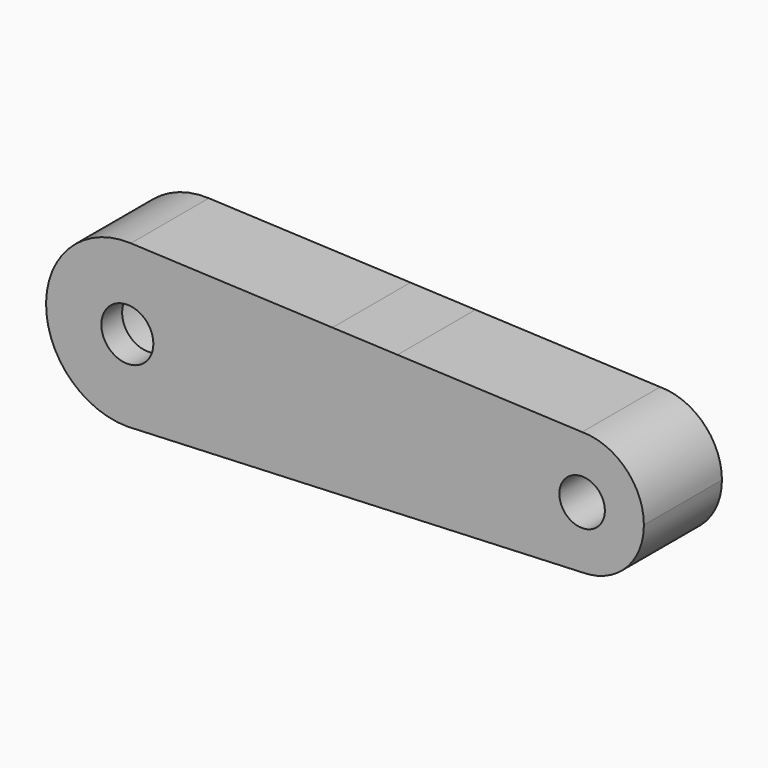
from build123d import *

# Parameters (mm, degrees)
F0_R     = 4.445
F1_DEPTH = 19.05
F3_DEPTH = 13.97
F4_R     = 5.08
F5_DEPTH = 5.08


with BuildPart() as f1:
    # F0 (on Front) → F1 (new body)
    with BuildSketch(Plane.XZ):
        with BuildLine():
            ThreePointArc((-124.9322268395, 28.7639294598), (-130.4980059639, 35.017678352), (-138.4710976488, 37.5705358593))
            ThreePointArc((-138.4710976488, 37.5705358593), (-155.0254015346, 22.0518028606), (-139.1540765762, 5.8352343242))
            Line((-139.1540765762, 5.8352343242), (-137.7946125004, 5.8935506507))
            ThreePointArc((-137.7946125004, 5.8935506507), (-130.1034423833, 8.6679321614), (-124.8131018813, 14.9019988847))
            Line((-124.8131018813, 14.9019988847), (-133.3336122029, 14.1704850261))
            ThreePointArc((-133.3336122029, 14.1704850261), (-148.6790765762, 21.7102343242), (-133.3336122029, 29.2499836224))
            Line((-133.3336122029, 29.2499836224), (-124.9322268395, 28.7639294598))
        make_face()
        with BuildLine():
            Line((-99.1008544222, 34.8894799677), (-99.1008544222, 35.8751666308))
            Line((-99.1008544222, 35.8751666308), (-138.4710976488, 37.5705358593))
            ThreePointArc((-138.4710976488, 37.5705358593), (-130.4980059639, 35.017678352), (-124.9322268395, 28.7639294598))
            Line((-124.9322268395, 28.7639294598), (-110.4319389367, 27.9250290893))
            ThreePointArc((-110.4319389367, 27.9250290893), (-105.7509869831, 33.0091720577), (-99.1008544222, 34.8894799677))
        make_face()
        with BuildLine():
            Line((-137.7946125004, 5.8935506507), (-99.0179549294, 7.5569357044))
            Line((-99.0179549294, 7.5569357044), (-99.1008544222, 9.4894799677))
            ThreePointArc((-99.1008544222, 9.4894799677), (-105.6044119808, 11.2810548255), (-110.273070294, 16.1503084588))
            Line((-110.273070294, 16.1503084588), (-124.8131018813, 14.9019988847))
            ThreePointArc((-124.8131018813, 14.9019988847), (-130.1034423833, 8.6679321614), (-137.7946125004, 5.8935506507))
        make_face()
        with BuildLine():
            ThreePointArc((-99.1008544222, 9.4894799677), (-96.8524942518, 9.6900849205), (-94.6751627721, 10.2855624017))
            ThreePointArc((-94.6751627721, 10.2855624017), (-88.6726167006, 14.9409036921), (-86.4008544222, 22.1894799677))
            Line((-86.4008544222, 22.1894799677), (-94.0208544222, 22.1894799677))
            ThreePointArc((-94.0208544222, 22.1894799677), (-95.5087519738, 18.5973775193), (-99.1008544222, 17.1094799677))
            Line((-99.1008544222, 17.1094799677), (-110.273070294, 16.1503084588))
            ThreePointArc((-110.273070294, 16.1503084588), (-105.6044119808, 11.2810548255), (-99.1008544222, 9.4894799677))
        make_face()
        with BuildLine():
            ThreePointArc((-86.4008544222, 22.1894799677), (-88.0348602906, 28.4211550137), (-92.5164093638, 33.0492720132))
            ThreePointArc((-92.5164093638, 33.0492720132), (-95.6824746143, 34.4207791419), (-99.1008544222, 34.8894799677))
            ThreePointArc((-99.1008544222, 34.8894799677), (-105.7509869831, 33.0091720577), (-110.4319389367, 27.9250290893))
            Line((-110.4319389367, 27.9250290893), (-99.1008544222, 27.2694799677))
            ThreePointArc((-99.1008544222, 27.2694799677), (-95.5087519738, 25.7815824161), (-94.0208544222, 22.1894799677))
            Line((-94.0208544222, 22.1894799677), (-86.4008544222, 22.1894799677))
        make_face()
        with BuildLine():
            Line((-99.0179549294, 7.5569357044), (-87.6442336226, 8.0448291746))
            Line((-87.6442336226, 8.0448291746), (-87.7530907655, 10.5824954495))
            Line((-87.7530907655, 10.5824954495), (-94.6751627721, 10.2855624017))
            ThreePointArc((-94.6751627721, 10.2855624017), (-96.8524942518, 9.6900849205), (-99.1008544222, 9.4894799677))
            Line((-99.1008544222, 9.4894799677), (-99.0179549294, 7.5569357044))
        make_face()
        with BuildLine():
            Line((-86.5101311345, 32.7906284679), (-86.4008544222, 35.3282767099))
            Line((-86.4008544222, 35.3282767099), (-99.1008544222, 35.8751666308))
            Line((-99.1008544222, 35.8751666308), (-99.1008544222, 34.8894799677))
            ThreePointArc((-99.1008544222, 34.8894799677), (-95.6824746143, 34.4207791419), (-92.5164093638, 33.0492720132))
            Line((-92.5164093638, 33.0492720132), (-86.5101311345, 32.7906284679))
        make_face()
        with BuildLine():
            ThreePointArc((-57.3392350777, 31.5344655517), (-54.0123637648, 33.2013955962), (-50.3357569569, 33.7752343242))
            Line((-50.3357569569, 33.7752343242), (-86.4008544222, 35.3282767099))
            Line((-86.4008544222, 35.3282767099), (-86.5101311345, 32.7906284679))
            Line((-86.5101311345, 32.7906284679), (-57.3392350777, 31.5344655517))
        make_face()
        with BuildLine():
            Line((-87.6442336226, 8.0448291746), (-50.3357569569, 9.6452343242))
            ThreePointArc((-50.3357569569, 9.6452343242), (-54.0132473827, 10.2193558039), (-57.3407458906, 11.8870802972))
            Line((-57.3407458906, 11.8870802972), (-87.7530907655, 10.5824954495))
            Line((-87.7530907655, 10.5824954495), (-87.6442336226, 8.0448291746))
        make_face()
        with BuildLine():
            ThreePointArc((-50.3357569569, 9.6452343242), (-41.8045136419, 13.1789910092), (-38.2707569569, 21.7102343242))
            ThreePointArc((-38.2707569569, 21.7102343242), (-41.8045136419, 30.2414776392), (-50.3357569569, 33.7752343242))
            ThreePointArc((-50.3357569569, 33.7752343242), (-54.0123637648, 33.2013955962), (-57.3392350777, 31.5344655517))
            ThreePointArc((-57.3392350777, 31.5344655517), (-62.4007569212, 21.7111620791), (-57.3407458906, 11.8870802972))
            ThreePointArc((-57.3407458906, 11.8870802972), (-54.0132473827, 10.2193558039), (-50.3357569569, 9.6452343242))
        make_face()
        with Locations((-50.3357569569, 21.7102343242)):
            Circle(F0_R, mode=Mode.SUBTRACT)
    extrude(amount=F1_DEPTH)

    # F2 (on face) → F3 (join)
    with BuildSketch(Plane.XZ.offset(19.05)):
        with BuildLine():
            ThreePointArc((-86.4008544222, 22.1894799677), (-88.6726167006, 14.9409036921), (-94.6751627721, 10.2855624017))
            Line((-94.6751627721, 10.2855624017), (-57.3407458906, 11.8870802972))
            ThreePointArc((-57.3407458906, 11.8870802972), (-62.4007569212, 21.7111620791), (-57.3392350777, 31.5344655517))
            Line((-57.3392350777, 31.5344655517), (-92.5164093638, 33.0492720132))
            ThreePointArc((-92.5164093638, 33.0492720132), (-88.0348602906, 28.4211550137), (-86.4008544222, 22.1894799677))
        make_face()
        with BuildLine():
            Line((-57.3407458906, 11.8870802972), (-94.6751627721, 10.2855624017))
            ThreePointArc((-94.6751627721, 10.2855624017), (-103.5704974557, 10.301995324), (-110.273070294, 16.1503084588))
            Line((-110.273070294, 16.1503084588), (-133.3336122029, 14.1704850261))
            ThreePointArc((-133.3336122029, 14.1704850261), (-148.6790765762, 21.7102343242), (-133.3336122029, 29.2499836224))
            Line((-133.3336122029, 29.2499836224), (-110.4319389367, 27.9250290893))
            ThreePointArc((-110.4319389367, 27.9250290893), (-102.5932909524, 34.3998397938), (-92.5164093638, 33.0492720132))
            Line((-92.5164093638, 33.0492720132), (-57.3392350777, 31.5344655517))
            ThreePointArc((-57.3392350777, 31.5344655517), (-54.0123637648, 33.2013955962), (-50.3357569569, 33.7752343242))
            Line((-50.3357569569, 33.7752343242), (-138.4710976488, 37.5705358593))
            ThreePointArc((-138.4710976488, 37.5705358593), (-155.0254015346, 22.0518028606), (-139.1540765762, 5.8352343242))
            Line((-139.1540765762, 5.8352343242), (-50.3357569569, 9.6452343242))
            ThreePointArc((-50.3357569569, 9.6452343242), (-54.0132473827, 10.2193558039), (-57.3407458906, 11.8870802972))
        make_face()
    extrude(amount=-F3_DEPTH)

    # F4 (on face) → F5 (join)
    with BuildSketch(Plane.XZ.offset(19.05)):
        with BuildLine():
            ThreePointArc((-133.3336122029, 29.2499836224), (-148.6790765762, 21.7102343242), (-133.3336122029, 14.1704850261))
            ThreePointArc((-133.3336122029, 14.1704850261), (-130.6052302168, 17.5098949424), (-129.6290765762, 21.7102343242))
            ThreePointArc((-129.6290765762, 21.7102343242), (-130.6052302168, 25.910573706), (-133.3336122029, 29.2499836224))
        make_face()
        with Locations((-139.1540765762, 21.7102343242)):
            Circle(F4_R, mode=Mode.SUBTRACT)
        with BuildLine():
            ThreePointArc((-129.6290765762, 21.7102343242), (-130.6052302168, 17.5098949424), (-133.3336122029, 14.1704850261))
            Line((-133.3336122029, 14.1704850261), (-99.1008544222, 17.1094799677))
            ThreePointArc((-99.1008544222, 17.1094799677), (-104.1808544222, 22.1894799677), (-99.1008544222, 27.2694799677))
            Line((-99.1008544222, 27.2694799677), (-133.3336122029, 29.2499836224))
            ThreePointArc((-133.3336122029, 29.2499836224), (-130.6052302168, 25.910573706), (-129.6290765762, 21.7102343242))
        make_face()
        with BuildLine():
            ThreePointArc((-99.1008544222, 27.2694799677), (-104.1808544222, 22.1894799677), (-99.1008544222, 17.1094799677))
            ThreePointArc((-99.1008544222, 17.1094799677), (-95.5087519738, 18.5973775193), (-94.0208544222, 22.1894799677))
            ThreePointArc((-94.0208544222, 22.1894799677), (-95.5087519738, 25.7815824161), (-99.1008544222, 27.2694799677))
        make_face()
    extrude(amount=-F5_DEPTH)


solid = f1.part
